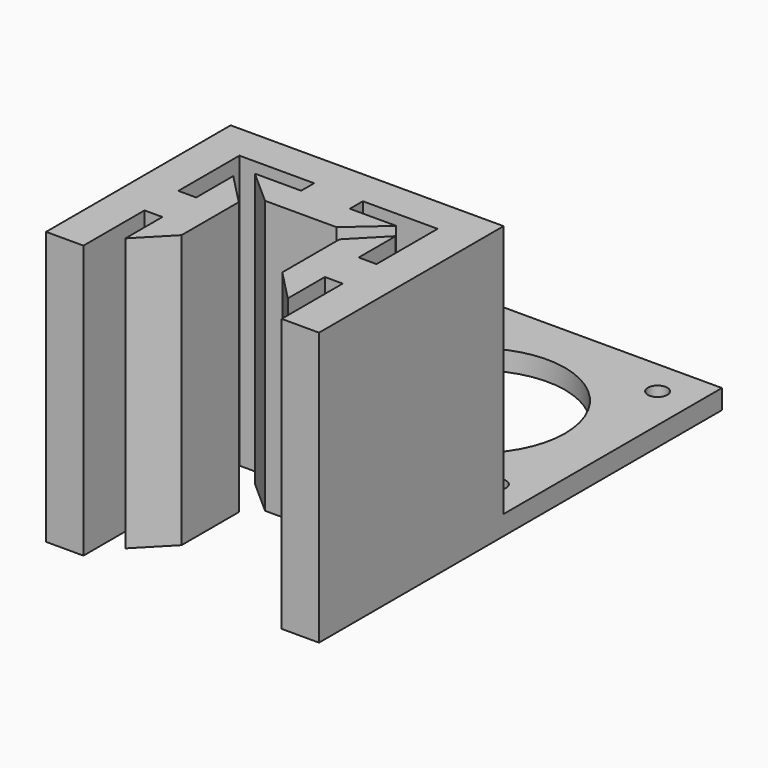
from build123d import *

# Parameters (mm, degrees)
F0_R     = 1.5
F0_R_2   = 13.6669430684
F1_DEPTH = 3
F2_DEPTH = 42


# Not quite as in the source:
# - a feature names something its author has since deleted; it is built from what else it names


with BuildPart() as f1:
    # F0 (on Top) → F1 (new body)
    with BuildSketch(Plane.XY):
        Polygon((21, 21), (-21, 21), (-21, -21), (-3.25, -21), (0, -21), (3.25, -21), (21, -21), align=None)
        with Locations((-15.5, -15.5)):
            Circle(F0_R, mode=Mode.SUBTRACT)
        with Locations((-15.5, 15.5)):
            Circle(F0_R, mode=Mode.SUBTRACT)
        Circle(F0_R_2, mode=Mode.SUBTRACT)
        with Locations((15.5, -15.5)):
            Circle(F0_R, mode=Mode.SUBTRACT)
        with Locations((15.5, 15.5)):
            Circle(F0_R, mode=Mode.SUBTRACT)
    extrude(amount=F1_DEPTH)

    # F0 (on Top) → F2 (join)
    with BuildSketch(Plane.XY):
        Polygon((12.5, -44.75), (15.25, -44.75), (15.25, -38.25), (12.5, -38.25), (12.5, -31.125), (7.75, -36), (7.75, -41.5), (7.75, -47), (12.5, -51.875), align=None)
        Polygon((-3.25, -21), (-21, -21), (-21, -26.5), (-21, -56.5), (-15.25, -56.5), (-15.25, -44.75), (-15.25, -38.25), (-15.25, -26.5), (-3.75, -26.5), (0, -26.5), (3.75, -26.5), (15.25, -26.5), (15.25, -38.25), (15.25, -44.75), (15.25, -56.5), (21, -56.5), (21, -26.5), (21, -21), (3.25, -21), (0, -21), align=None)
        Polygon((0, -26.5), (-3.75, -26.5), (-3.75, -29), (-10.875, -29), (-5.5, -33.75), (0, -33.75), (5.5, -33.75), (10.875, -29), (3.75, -29), (3.75, -26.5), align=None)
        Polygon((-15.25, -38.25), (-15.25, -44.75), (-12.5, -44.75), (-12.5, -51.875), (-7.75, -47), (-7.75, -41.5), (-7.75, -36), (-12.5, -31.125), (-12.5, -38.25), align=None)
    extrude(amount=F2_DEPTH)


solid = f1.part
